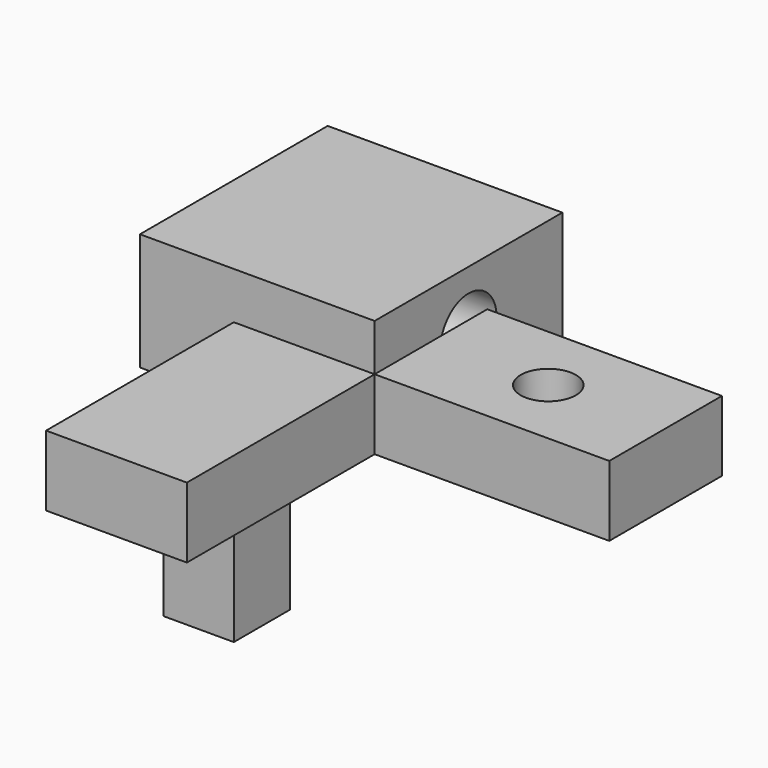
from build123d import *

# Parameters (mm, degrees)
F0_W     = 100
F0_H     = 60
F0_R     = 11.7517787986
F1_DEPTH = 30
F2_W     = 60
F2_H     = 100
F3_DEPTH = 30
F4_W     = 100
F4_H     = 100
F5_DEPTH = 50
F6_R     = 15
F7_DEPTH = 100
F2_W_2   = 30
F2_H_2   = 30
F8_DEPTH = 90


with BuildPart() as f1:
    # F0 (on Top) → F1 (new body)
    with BuildSketch(Plane.XY):
        with Locations((50, 30)):
            Rectangle(F0_W, F0_H)
        with Locations((50, 30)):
            Circle(F0_R, mode=Mode.SUBTRACT)
    extrude(amount=F1_DEPTH)


with BuildPart() as f3:
    # F2 (on Top) → F3 (new body)
    with BuildSketch(Plane.XY):
        with Locations((-30, -50)):
            Rectangle(F2_W, F2_H)
    extrude(amount=F3_DEPTH)


with BuildPart() as f5:
    # F4 (on Top) → F5 (new body)
    with BuildSketch(Plane.XY):
        with Locations((-50, 50)):
            Rectangle(F4_W, F4_H)
    extrude(amount=F5_DEPTH)

    # F6 (on face) → F7 (cut, through all)
    with BuildSketch(Plane(origin=(-100, 0, 0), x_dir=(0, -1, 0), z_dir=(-1, 0, 0))):
        with Locations((-50, 25)):
            Circle(F6_R)
    extrude(amount=-F7_DEPTH, mode=Mode.SUBTRACT)

    # F2 (on Top) → F8 (join)
    with BuildSketch(Plane.XY):
        with Locations((-75, 15)):
            Rectangle(F2_W_2, F2_H_2)
    extrude(amount=-F8_DEPTH)


solid = Compound([f1.part, f3.part, f5.part])
